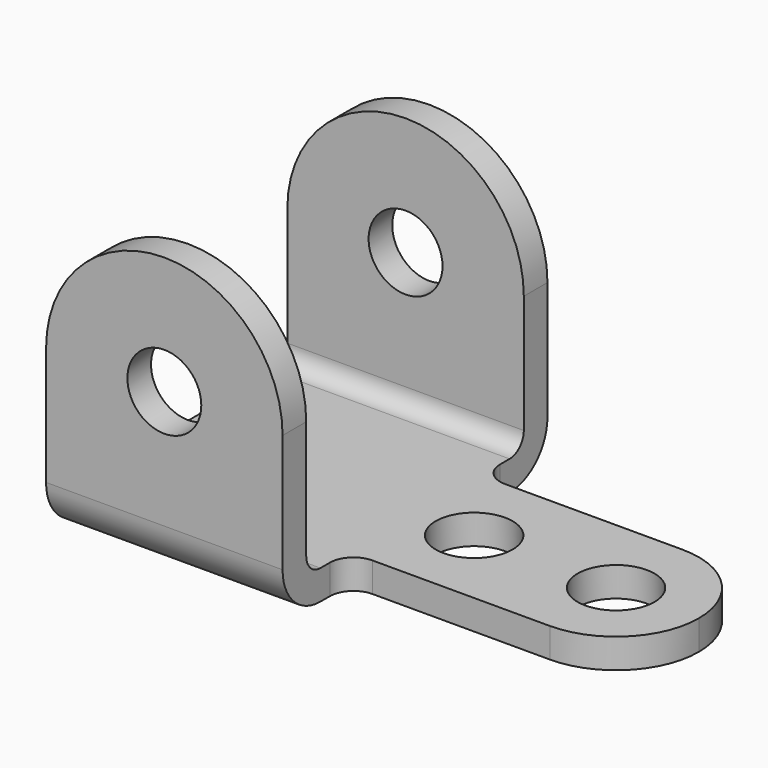
from build123d import *

# Parameters (mm, degrees)
F1_DEPTH  = 63.5
F3_DEPTH  = 7.9375
F5_DEPTH  = 7.9375
F7_DEPTH  = 7.9375
F8_R      = 6.35
F9_R      = 9.92251
F10_DEPTH = 88.901
F11_R     = 10.3251
F12_DEPTH = 7.9385


with BuildPart() as f1:
    # F0 (on Right) → F1 (new body)
    with BuildSketch(Plane.YZ):
        with BuildLine():
            Line((-36.5125, 44.45), (-44.45, 44.45))
            Line((-44.45, 44.45), (-44.45, 12.7))
            ThreePointArc((-44.45, 12.7), (-40.7302561211, 3.7197438789), (-31.75, 0))
            Line((-31.75, 0), (0, 0))
            Line((0, 0), (0, 7.9375))
            Line((0, 7.9375), (-31.75, 7.9375))
            ThreePointArc((-31.75, 7.9375), (-35.1175960454, 9.3324039546), (-36.5125, 12.7))
            Line((-36.5125, 12.7), (-36.5125, 44.45))
        make_face()
        with BuildLine():
            Line((0, 7.9375), (0, 0))
            Line((0, 0), (31.75, 0))
            ThreePointArc((31.75, 0), (40.7302561211, 3.7197438789), (44.45, 12.7))
            Line((44.45, 12.7), (44.45, 44.45))
            Line((44.45, 44.45), (36.5125, 44.45))
            Line((36.5125, 44.45), (36.5125, 12.7))
            ThreePointArc((36.5125, 12.7), (35.1175960454, 9.3324039546), (31.75, 7.9375))
            Line((31.75, 7.9375), (0, 7.9375))
        make_face()
    extrude(amount=F1_DEPTH)

    # F2 (on face) → F3 (join, through all)
    with BuildSketch(Plane.XZ.offset(44.45)):
        with BuildLine():
            Line((0, 44.45), (63.5, 44.45))
            ThreePointArc((63.5, 44.45), (31.75, 76.2), (0, 44.45))
        make_face()
    extrude(amount=-F3_DEPTH)

    # F4 (on face) → F5 (join, through all)
    with BuildSketch(Plane(origin=(0, 44.45, 0), x_dir=(-1, 0, 0), z_dir=(0, 1, 0))):
        with BuildLine():
            ThreePointArc((0, 44.45), (-31.75, 76.2), (-63.5, 44.45))
            Line((-63.5, 44.45), (0, 44.45))
        make_face()
    extrude(amount=-F5_DEPTH)

    # F6 (on face) → F7 (join, through all)
    with BuildSketch(Plane(origin=(0, 0, 0), x_dir=(1, 0, 0), z_dir=(0, 0, -1))):
        with BuildLine():
            Line((63.5, 22.225), (63.5, -22.225))
            Line((63.5, -22.225), (117.475, -22.225))
            ThreePointArc((117.475, -22.225), (133.1904482119, -15.7154482119), (139.7, 0))
            ThreePointArc((139.7, 0), (133.1904482119, 15.7154482119), (117.475, 22.225))
            Line((117.475, 22.225), (63.5, 22.225))
        make_face()
    extrude(amount=-F7_DEPTH)

    # F8
    f8_edges = [f1.edges().sort_by_distance(p)[0] for p in [
        (63.5, -22.225, 3.96875),
        (63.5, 22.225, 3.96875),
    ]]
    fillet(f8_edges, radius=F8_R)

    # F9 (on face) → F10 (cut, through all)
    with BuildSketch(Plane.XZ.offset(44.45)):
        with Locations((31.75, 44.45)):
            Circle(F9_R)
    extrude(amount=-F10_DEPTH, mode=Mode.SUBTRACT)

    # F11 (on face) → F12 (cut, through all)
    with BuildSketch(Plane.XY.offset(7.9375)):
        with Locations((117.475, 0)):
            Circle(F11_R)
        with Locations((79.375, 0)):
            Circle(F11_R)
    extrude(amount=-F12_DEPTH, mode=Mode.SUBTRACT)


solid = f1.part
